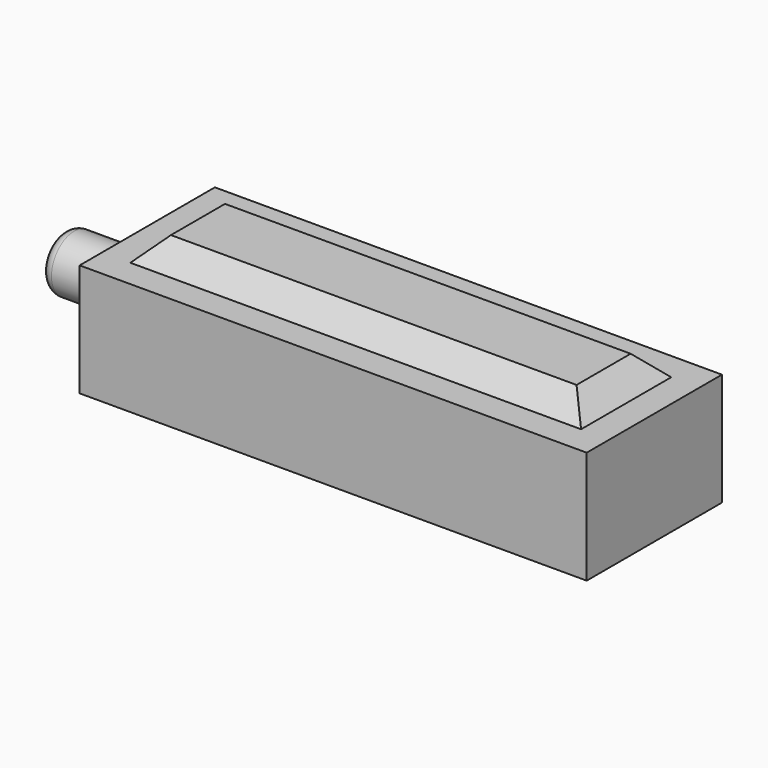
from build123d import *

# Parameters (mm, degrees)
F0_W     = 114.3
F0_H     = 38.1
F1_DEPTH = 25.4
F2_R     = 6.35
F3_DEPTH = 19.05
F4_R     = 2.54
F5_W     = 101.6
F5_H     = 25.4
F6_DEPTH = 5.08
F7_SIZE  = 5.07999
F8_W     = 76.2
F8_H     = 12.7
F9_DEPTH = 12.7
F10_R    = 6.34999


# Not quite as in the source:
# - a fillet or chamfer is up to 0.001 mm smaller than in the source, because OpenCascade refuses the exact size


with BuildPart() as f1:
    # F0 (on Top) → F1 (new body)
    with BuildSketch(Plane.XY):
        Rectangle(F0_W, F0_H)
    extrude(amount=F1_DEPTH)

    # F2 (on face) → F3 (join)
    with BuildSketch(Plane(origin=(-57.15, 0, 0), x_dir=(0, -1, 0), z_dir=(-1, 0, 0))):
        with Locations((0, 12.7)):
            Circle(F2_R)
    extrude(amount=F3_DEPTH)

    # F4
    f4_edges = [f1.edges().sort_by_distance(p)[0] for p in [
        (-76.2, 6.35, 12.7),
    ]]
    fillet(f4_edges, radius=F4_R)

    # F5 (on face) → F6 (join)
    with BuildSketch(Plane.XY.offset(25.4)):
        Rectangle(F5_W, F5_H)
    extrude(amount=F6_DEPTH)

    # F7 (size 5.08 in the source; OpenCascade refuses exactly that, so slightly less here)
    f7_edges = [f1.edges().sort_by_distance(p)[0] for p in [
        (0, -12.7, 30.48),
        (-50.8, 0, 30.48),
        (50.8, 0, 30.48),
        (0, 12.7, 30.48),
    ]]
    chamfer(f7_edges, length=F7_SIZE)

    # F8 (on face) → F9 (cut)
    with BuildSketch(Plane(origin=(0, 0, 0), x_dir=(1, 0, 0), z_dir=(0, 0, -1))):
        Rectangle(F8_W, F8_H)
    extrude(amount=-F9_DEPTH, mode=Mode.SUBTRACT)

    # F10 (radius 6.35 in the source; OpenCascade refuses exactly that, so slightly less here)
    f10_edges = [f1.edges().sort_by_distance(p)[0] for p in [
        (0, 6.35, 12.7),
        (0, -6.35, 12.7),
    ]]
    fillet(f10_edges, radius=F10_R)


solid = f1.part
